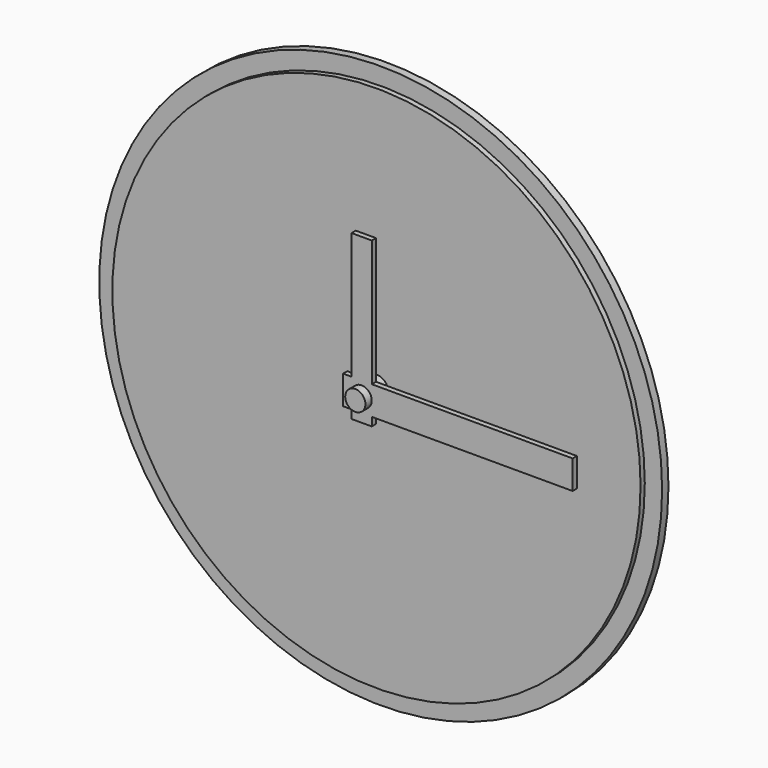
from build123d import *

# Parameters (mm, degrees)
F0_R      = 106.500216
F1_DEPTH  = 5
F2_R      = 4.595157
F3_DEPTH  = 5
F4_W      = 3.217991
F4_H      = 10.860724
F4_W_2    = 7.642738
F4_H_2    = 47.867635
F4_W_3    = 76.025058
F4_H_3    = 3.217992
F5_DEPTH  = 2
F6_R      = 106.500216
F6_R_2    = 99.941282
F7_DEPTH  = 2
F8_W      = 75.220562
F8_H      = 89.701534
F9_DEPTH  = 13
F10_W     = 53.499122
F10_H     = 30.570925
F11_DEPTH = 3
F12_R     = 6.718922
F13_DEPTH = 2
F14_R     = 3.625825
F15_DEPTH = 7
F16_W     = 36.604659
F16_H     = 7.240483
F17_DEPTH = 4
F18_R     = 3.821369
F19_DEPTH = 3
F20_R     = 100.37101
F20_W     = 75.220562
F20_H     = 89.701534
F21_DEPTH = 2


with BuildPart() as f1:
    # F0 (on Front) → F1 (new body)
    with BuildSketch(Plane.XZ):
        Circle(F0_R)
    extrude(amount=F1_DEPTH)

    # F2 (on face) → F3 (join)
    with BuildSketch(Plane.XZ.offset(5)):
        Circle(F2_R)
    extrude(amount=F3_DEPTH)

    # F4 (on face) → F5 (join)
    with BuildSketch(Plane.XZ.offset(10)):
        with BuildLine():
            Line((79.846427, 5.430362), (3.821369, 5.430362))
            Line((3.821369, 5.430362), (3.821369, 2.551981))
            ThreePointArc((3.821369, 2.551981), (4.397457, 1.333356), (4.595157, 0))
            ThreePointArc((4.595157, 0), (4.397457, -1.333356), (3.821369, -2.551981))
            Line((3.821369, -2.551981), (3.821369, -5.430362))
            Line((3.821369, -5.430362), (79.846427, -5.430362))
            Line((79.846427, -5.430362), (79.846427, 5.430362))
        make_face()
        with Locations((-5.430364, 0)):
            Rectangle(F4_W, F4_H)
        with Locations((0, 29.364179)):
            Rectangle(F4_W_2, F4_H_2)
        Rectangle(F4_W_2, F4_H)
        with Locations((41.833898, 0)):
            Rectangle(F4_W_3, F4_H)
        with Locations((0, -7.039358)):
            Rectangle(F4_W_2, F4_H_3)
    extrude(amount=F5_DEPTH)

    # F6 (on face) → F7 (cut)
    with BuildSketch(Plane.XZ.offset(5)):
        Circle(F6_R)
        Circle(F6_R_2, mode=Mode.SUBTRACT)
    extrude(amount=-F7_DEPTH, mode=Mode.SUBTRACT)

    # F8 (on face) → F9 (join)
    with BuildSketch(Plane(origin=(0, 0, 0), x_dir=(-1, 0, 0), z_dir=(0, 1, 0))):
        Rectangle(F8_W, F8_H)
    extrude(amount=F9_DEPTH)

    # F10 (on face) → F11 (cut)
    with BuildSketch(Plane(origin=(0, 13, 0), x_dir=(-1, 0, 0), z_dir=(0, 1, 0))):
        with Locations((0, -9.855101)):
            Rectangle(F10_W, F10_H)
    extrude(amount=-F11_DEPTH, mode=Mode.SUBTRACT)

    # F12 (on face) → F13 (join)
    with BuildSketch(Plane(origin=(0, 10, 0), x_dir=(-1, 0, 0), z_dir=(0, 1, 0))):
        with Locations((13.717563, -5.033229)):
            Circle(F12_R)
    extrude(amount=F13_DEPTH)

    # F14 (on face) → F15 (cut)
    with BuildSketch(Plane(origin=(0, 13, 0), x_dir=(-1, 0, 0), z_dir=(0, 1, 0))):
        with Locations((0, 30.3698)):
            Circle(F14_R)
    extrude(amount=-F15_DEPTH, mode=Mode.SUBTRACT)

    # F16 (on face) → F17 (join)
    with BuildSketch(Plane(origin=(0, 10, 0), x_dir=(-1, 0, 0), z_dir=(0, 1, 0))):
        with Locations((0.402248, -18.302331)):
            Rectangle(F16_W, F16_H)
    extrude(amount=F17_DEPTH)

    # F18 (on face) → F19 (join)
    with BuildSketch(Plane.XZ.offset(12)):
        Circle(F18_R)
    extrude(amount=F19_DEPTH)

    # F20 (on face) → F21 (join)
    with BuildSketch(Plane(origin=(0, 0, 0), x_dir=(-1, 0, 0), z_dir=(0, 1, 0))):
        Circle(F20_R)
        Rectangle(F20_W, F20_H, mode=Mode.SUBTRACT)
    extrude(amount=F21_DEPTH)


solid = f1.part
